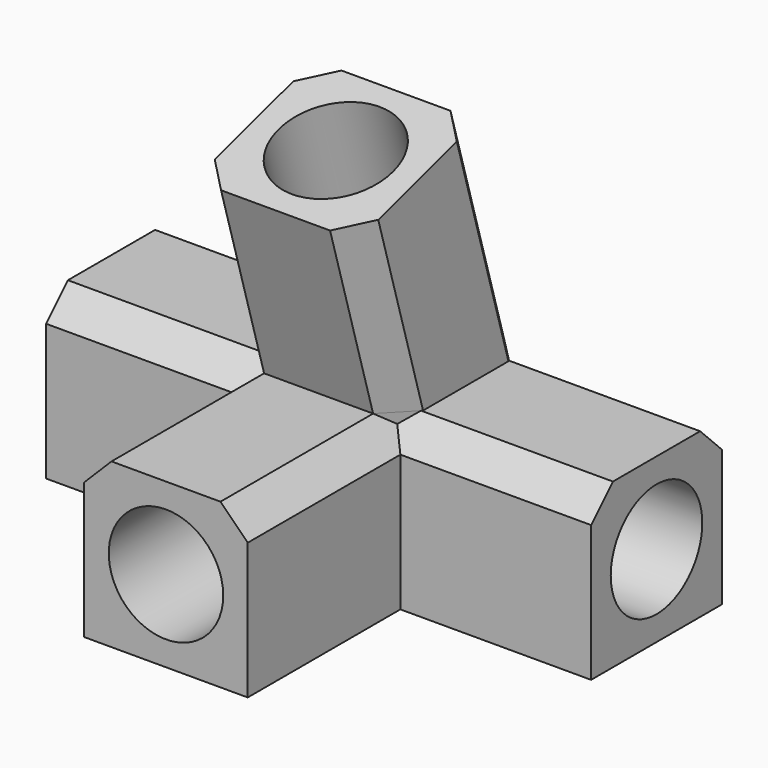
from build123d import *

# Parameters (mm, degrees)
F0_W          = 100
F0_H          = 30
F1_DEPTH      = 30
F3_R          = 10.5
F4_DEPTH      = 100
F5_W          = 30
F5_H          = 30
F6_DEPTH      = 35
F2_W          = 30
F2_H          = 30
F7_DEPTH      = 35
F9_DEPTH      = 5
F10_DEPTH     = 35
F11_DEPTH     = 30
F12_DEPTH     = 5
F13_R         = 10.5
F14_DEPTH     = 50
F15_R         = 10.5
F16_DEPTH     = 50
F17_T4_DEPTH  = 78.1749423251
F17_T9_DEPTH  = 78.1749423251
F17_T14_DEPTH = 60.7168298797
F17_T19_DEPTH = 60.7168298797
F18_T4_DEPTH  = 52.8584149398
F18_T9_DEPTH  = 60.7168298797
F18_T15_DEPTH = 60.7168298797
F18_T21_DEPTH = 60.7168298797
F18_T27_DEPTH = 60.7168298797
F18_T33_DEPTH = 52.8584149398


# Not quite as in the source:
# - a fillet or chamfer that OpenCascade refuses, or shapes differently, is made with other operations: its cross-section is extruded or revolved along the edge and cut away or added


with BuildPart() as f1:
    # F0 (on Top) → F1 (new body)
    with BuildSketch(Plane.XY):
        Rectangle(F0_W, F0_H)
    extrude(amount=F1_DEPTH)

    # F3 (on face) → F4 (cut)
    with BuildSketch(Plane(origin=(-50, 0, 0), x_dir=(0, -1, 0), z_dir=(-1, 0, 0))):
        with Locations((0, 15)):
            Circle(F3_R)
    extrude(amount=-F4_DEPTH, mode=Mode.SUBTRACT)

    # F5 (on face) → F6 (join)
    with BuildSketch(Plane.XZ.offset(15)):
        with Locations((0, 15)):
            Rectangle(F5_W, F5_H)
    extrude(amount=F6_DEPTH)

    # F2 (on face) → F7 (join)
    with BuildSketch(Plane.XY.offset(30)):
        Rectangle(F2_W, F2_H)
    extrude(amount=F7_DEPTH)

    # F8 (on face) → F9 (join)
    with BuildSketch(Plane(origin=(-15, 0, 0), x_dir=(0, -1, 0), z_dir=(-1, 0, 0))):
        Polygon((15, 65), (15, 30), (24.8667589854, 63.5804566247), (-2.7490875563, 71.6946673709), (-4.7161444721, 65), align=None)
        Polygon((-15, 30), (15, 30), (15, 65), (-4.7161444721, 65), align=None)
    extrude(amount=F9_DEPTH)

    # F10 (cut, through all): a face of the model
    f10_faces = [f1.faces().sort_by_distance(p)[0] for p in [
        (0, 0, 65),
    ]]
    extrude(f10_faces, amount=-F10_DEPTH, mode=Mode.SUBTRACT)

    # F8 (on face) → F11 (join)
    with BuildSketch(Plane(origin=(-15, 0, 0), x_dir=(0, -1, 0), z_dir=(-1, 0, 0))):
        Polygon((-15, 30), (15, 30), (15, 65), (-4.7161444721, 65), align=None)
        Polygon((15, 65), (15, 30), (24.8667589854, 63.5804566247), (-2.7490875563, 71.6946673709), (-4.7161444721, 65), align=None)
    extrude(amount=-F11_DEPTH)

    # F12 (cut): a face of the model
    f12_faces = [f1.faces().sort_by_distance(p)[0] for p in [
        (-20, -5.0118640534, 48.8916696379),
    ]]
    extrude(f12_faces, amount=-F12_DEPTH, mode=Mode.SUBTRACT)

    # F13 (on face) → F14 (cut)
    with BuildSketch(Plane.XZ.offset(50)):
        with Locations((0, 15)):
            Circle(F13_R)
    extrude(amount=-F14_DEPTH, mode=Mode.SUBTRACT)

    # F15 (on face) → F16 (cut)
    with BuildSketch(Plane(origin=(0, -19.1730464608, 65.2534085396), x_dir=(1, 0, 0), z_dir=(0, -0.2819073996, 0.9594416178))):
        with Locations((0, 8.4572219875)):
            Circle(F15_R)
    extrude(amount=-F16_DEPTH, mode=Mode.SUBTRACT)

    # F17: chamfer of 5 on 4 edges, made by hand


with BuildPart() as f17_tool2:
    # F17_s3 → F17_t4 (new body)
    with BuildSketch(Plane(origin=(0, -22.7979287792, 77.5903069724), x_dir=(1, 0, 0), z_dir=(0, 0.2819073996, -0.9594416178))):
        Polygon((-10, -22.8488462553), (-15, -17.8488462553), (-15, -22.8488462553), align=None)
    extrude(amount=F17_T4_DEPTH)

    split(bisect_by=Plane.XY.offset(30), keep=Keep.TOP)


with BuildPart() as f1_1:
    add(f1.part)

    # F17_t1: cut F17_tool2
    add(f17_tool2.part, mode=Mode.SUBTRACT)


with BuildPart() as f17_tool7:
    # F17_s8 → F17_t9 (new body)
    with BuildSketch(Plane(origin=(0, -22.7979287792, 77.5903069724), x_dir=(1, 0, 0), z_dir=(0, 0.2819073996, -0.9594416178))):
        Polygon((15, -17.8488462553), (10, -22.8488462553), (15, -22.8488462553), align=None)
    extrude(amount=F17_T9_DEPTH)

    split(bisect_by=Plane.XY.offset(30), keep=Keep.TOP)


with BuildPart() as f1_2:
    add(f1_1.part)

    # F17_t6: cut F17_tool7
    add(f17_tool7.part, mode=Mode.SUBTRACT)


with BuildPart() as f17_tool12:
    # F17_s13 → F17_t14 (new body)
    with BuildSketch(Plane(origin=(0, -5.6814051569, 19.3360534821), x_dir=(1, 0, 0), z_dir=(0, -0.2819073996, 0.9594416178))):
        Polygon((15, -0.9344022802), (10, -5.9344022802), (15, -5.9344022802), align=None)
    extrude(amount=F17_T14_DEPTH)

    split(bisect_by=Plane.XY.offset(30), keep=Keep.TOP)


with BuildPart() as f1_3:
    add(f1_2.part)

    # F17_t11: cut F17_tool12
    add(f17_tool12.part, mode=Mode.SUBTRACT)


with BuildPart() as f17_tool17:
    # F17_s18 → F17_t19 (new body)
    with BuildSketch(Plane(origin=(0, -5.6814051569, 19.3360534821), x_dir=(1, 0, 0), z_dir=(0, -0.2819073996, 0.9594416178))):
        Polygon((-10, -5.9344022802), (-15, -0.9344022802), (-15, -5.9344022802), align=None)
    extrude(amount=F17_T19_DEPTH)

    split(bisect_by=Plane.XY.offset(30), keep=Keep.TOP)


with BuildPart() as f1_4:
    add(f1_3.part)

    # F17_t16: cut F17_tool17
    add(f17_tool17.part, mode=Mode.SUBTRACT)

    # F18: chamfer of 5 on 6 edges, made by hand


with BuildPart() as f18_tool2:
    # F18_s3 → F18_t4 (new body)
    with BuildSketch(Plane.YZ.offset(62.8584149398)):
        Polygon((10, 30), (15, 25), (15, 30), align=None)
    extrude(amount=-F18_T4_DEPTH)

    split(bisect_by=Plane(origin=(16.4244231276, 15.7582750978, 4.6301664136), x_dir=(-0.6923221184, 0.7215885839, 0), z_dir=(0.7071067812, 0.6784276741, 0.1993386339)), keep=Keep.TOP)


with BuildPart() as f1_5:
    add(f1_4.part)

    # F18_t1: cut F18_tool2
    add(f18_tool2.part, mode=Mode.SUBTRACT)


with BuildPart() as f18_tool7:
    # F18_s8 → F18_t9 (new body)
    with BuildSketch(Plane.YZ.offset(-2.1415850602)):
        Polygon((-10, 30), (-15, 25), (-15, 30), align=None)
    extrude(amount=-F18_T9_DEPTH)

    split(bisect_by=Plane(origin=(-7.9672011401, -7.6440643516, -2.2460129554), x_dir=(0.6923221184, -0.7215885839, 0), z_dir=(-0.7071067812, -0.6784276741, -0.1993386339)), keep=Keep.TOP)

    split(bisect_by=Plane(origin=(-20, 0, 20), x_dir=(0, 1, 0), z_dir=(-0.7071067812, 0, 0.7071067812)), keep=Keep.TOP)


with BuildPart() as f1_6:
    add(f1_5.part)

    # F18_t6: cut F18_tool7
    add(f18_tool7.part, mode=Mode.SUBTRACT)


with BuildPart() as f18_tool13:
    # F18_s14 → F18_t15 (new body)
    with BuildSketch(Plane.YZ.offset(2.1415850602)):
        Polygon((-15, 25), (-10, 30), (-15, 30), align=None)
    extrude(amount=F18_T15_DEPTH)

    split(bisect_by=Plane(origin=(7.9672011401, -7.6440643516, -2.2460129554), x_dir=(0.6923221184, 0.7215885839, 0), z_dir=(0.7071067812, -0.6784276741, -0.1993386339)), keep=Keep.TOP)

    split(bisect_by=Plane(origin=(20, 0, 20), x_dir=(0, 1, 0), z_dir=(0.7071067812, 0, 0.7071067812)), keep=Keep.TOP)


with BuildPart() as f1_7:
    add(f1_6.part)

    # F18_t12: cut F18_tool13
    add(f18_tool13.part, mode=Mode.SUBTRACT)


with BuildPart() as f18_tool19:
    # F18_s20 → F18_t21 (new body)
    with BuildSketch(Plane.XZ.offset(2.1415850602)):
        Polygon((-10, 30), (-15, 25), (-15, 30), align=None)
    extrude(amount=F18_T21_DEPTH)

    split(bisect_by=Plane(origin=(-7.9672011401, -7.6440643516, -2.2460129554), x_dir=(0.6923221184, -0.7215885839, 0), z_dir=(-0.7071067812, -0.6784276741, -0.1993386339)), keep=Keep.TOP)

    split(bisect_by=Plane(origin=(0, -20, 20), x_dir=(1, 0, 0), z_dir=(0, -0.7071067812, 0.7071067812)), keep=Keep.TOP)


with BuildPart() as f1_8:
    add(f1_7.part)

    # F18_t18: cut F18_tool19
    add(f18_tool19.part, mode=Mode.SUBTRACT)


with BuildPart() as f18_tool25:
    # F18_s26 → F18_t27 (new body)
    with BuildSketch(Plane.XZ.offset(2.1415850602)):
        Polygon((10, 30), (15, 25), (15, 30), align=None)
    extrude(amount=F18_T27_DEPTH)

    split(bisect_by=Plane(origin=(7.9672011401, -7.6440643516, -2.2460129554), x_dir=(0.6923221184, 0.7215885839, 0), z_dir=(0.7071067812, -0.6784276741, -0.1993386339)), keep=Keep.TOP)

    split(bisect_by=Plane(origin=(0, -20, 20), x_dir=(1, 0, 0), z_dir=(0, -0.7071067812, 0.7071067812)), keep=Keep.TOP)


with BuildPart() as f1_9:
    add(f1_8.part)

    # F18_t24: cut F18_tool25
    add(f18_tool25.part, mode=Mode.SUBTRACT)


with BuildPart() as f18_tool31:
    # F18_s32 → F18_t33 (new body)
    with BuildSketch(Plane.YZ.offset(-62.8584149398)):
        Polygon((10, 30), (15, 25), (15, 30), align=None)
    extrude(amount=F18_T33_DEPTH)

    split(bisect_by=Plane(origin=(-16.4244231276, 15.7582750978, 4.6301664136), x_dir=(-0.6923221184, -0.7215885839, 0), z_dir=(-0.7071067812, 0.6784276741, 0.1993386339)), keep=Keep.TOP)


with BuildPart() as f1_10:
    add(f1_9.part)

    # F18_t30: cut F18_tool31
    add(f18_tool31.part, mode=Mode.SUBTRACT)


solid = f1_10.part
